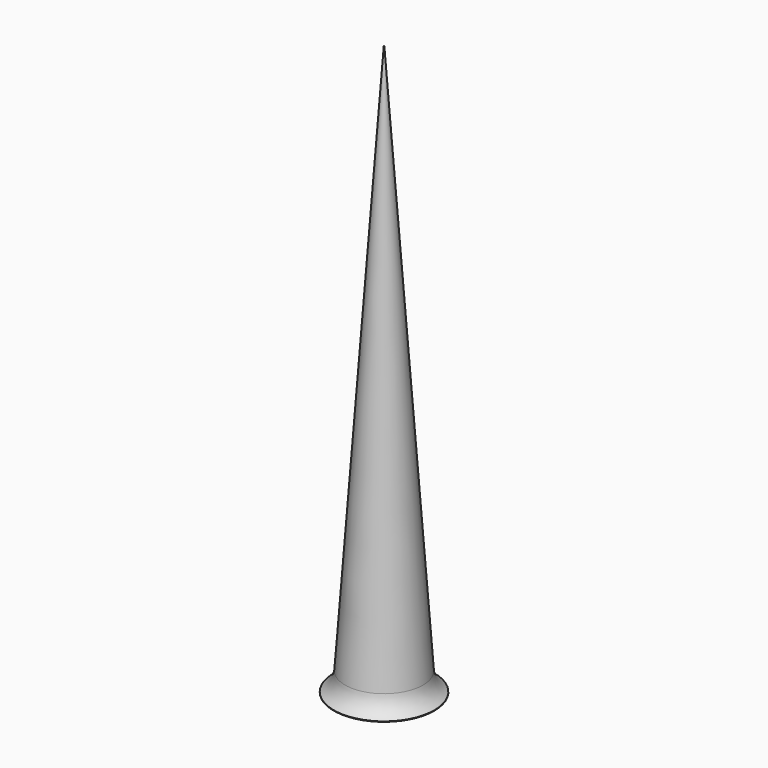
from build123d import *

# Parameters (mm, degrees)
F0_R     = 85
F2_R     = 0.5
F4_R     = 105.9677495378
F5_DEPTH = 1


# Not quite as in the source:
# - a fillet or chamfer that OpenCascade refuses, or shapes differently, is made with other operations: its cross-section is extruded or revolved along the edge and cut away or added


with BuildPart() as f3:
    # F0 (on Top) → F3 section 0
    with BuildSketch(Plane.XY):
        Circle(F0_R)
    # F2 (on offset) → F3 section 1
    with BuildSketch(Plane.XY.offset(1200)):
        Circle(F2_R)
    loft()

    # F4 (on Top) → F5 (join)
    with BuildSketch(Plane.XY):
        Circle(F4_R)
    extrude(amount=F5_DEPTH)

    # F6: fillet of radius 50 on 1 edges, made by hand


with BuildPart() as f6_tool2:
    # F6_s3 → F6_t4 (revolve)
    with BuildSketch(Plane.XZ):
        with BuildLine():
            ThreePointArc((105.9675408797, 0.999658735), (89.3230206235, 17.6878237287), (82.1725940934, 40.1468153769))
            Line((82.1725940934, 40.1468153769), (77.1847958314, 39.7955912493))
            ThreePointArc((77.1847958314, 39.7955912493), (78.5634899573, 20.2221976094), (79.9417850713, 0.6487758724))
            Line((79.9417850713, 0.6487758724), (84.9295833333, -4.0001489868))
            ThreePointArc((84.9295833333, -4.0001489868), (95.4485621065, -4.0001489868), (103.3592372963, -3.2662810568))
            Line((103.3592372963, -3.2662810568), (105.9675408797, 0.999658735))
        make_face()
    revolve(axis=Axis((0, 0, 1), (0, 0, 1)))

    split(bisect_by=Plane.XY, keep=Keep.TOP)


with BuildPart() as f3_1:
    add(f3.part)

    # F6_t1: union F6_tool2
    add(f6_tool2.part)


solid = f3_1.part
